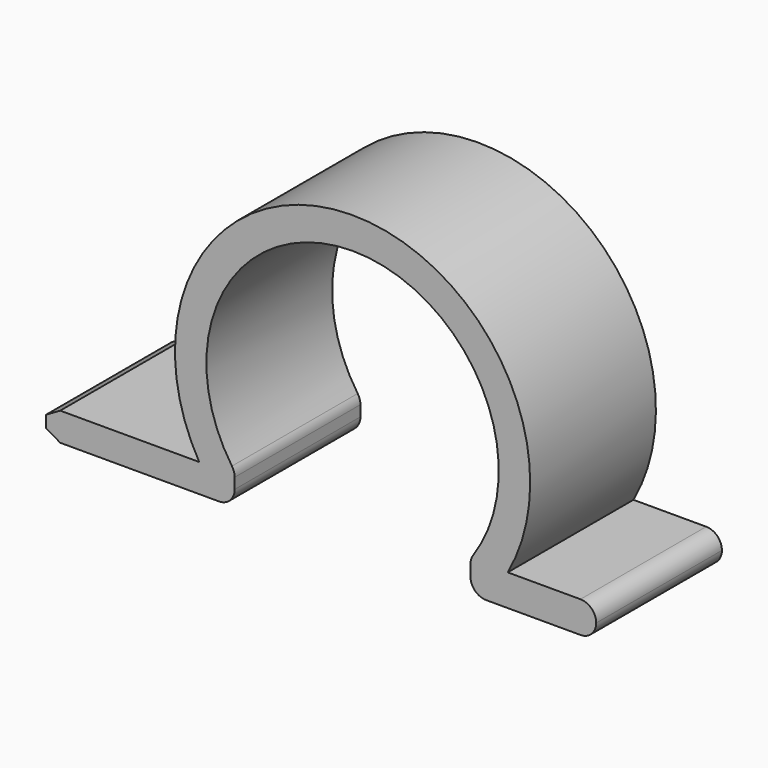
from build123d import *

# Parameters (mm, degrees)
F1_DEPTH   = 12.7
F2_SIZE2   = 0.6599113577
F2_SIZE    = 1.143
F2_2_SIZE2 = 0.6599113577
F2_2_SIZE  = 1.143
F3_R       = 1.26999


# Not quite as in the source:
# - a fillet or chamfer is up to 0.001 mm smaller than in the source, because OpenCascade refuses the exact size


with BuildPart() as f1:
    # F0 (on Front) → F1 (new body)
    with BuildSketch(Plane.XZ):
        with BuildLine():
            Line((0, 2.286), (0, 0))
            Line((0, 0), (15.24, 0))
            Line((15.24, 0), (15.24, 2.54))
            ThreePointArc((15.24, 2.54), (24.765, 21.336682776), (34.29, 2.54))
            Line((34.29, 2.54), (34.29, 0))
            Line((34.29, 0), (44.45, 0))
            Line((44.45, 0), (44.45, 2.54))
            Line((44.45, 2.54), (37.3021676826, 2.54))
            ThreePointArc((37.3021676826, 2.54), (24.6187816105, 23.8759379026), (12.3727573659, 2.286))
            Line((12.3727573659, 2.286), (0, 2.286))
        make_face()
    extrude(amount=F1_DEPTH)

    # F2
    f2_edges = [f1.edges().sort_by_distance(p)[0] for p in [
        (0, -6.35, 0),
    ]]
    f2_side = f1.faces().sort_by_distance((7.62, -6.35, 0))[0]
    chamfer(f2_edges, length=F2_SIZE, length2=F2_SIZE2, reference=f2_side)

    # F2#2
    f2_2_edges = [f1.edges().sort_by_distance(p)[0] for p in [
        (0, -6.35, 2.286),
    ]]
    f2_2_side = f1.faces().sort_by_distance((6.186379, -6.35, 2.286))[0]
    chamfer(f2_2_edges, length=F2_2_SIZE, length2=F2_2_SIZE2, reference=f2_2_side)

    # F3 (radius 1.27 in the source; OpenCascade refuses exactly that, so slightly less here)
    f3_edges = [f1.edges().sort_by_distance(p)[0] for p in [
        (44.45, -6.35, 2.54),
        (44.45, -6.35, 0),
        (34.29, -6.35, 0),
        (34.29, -6.35, 2.54),
        (15.24, -6.35, 2.54),
        (15.24, -6.35, 0),
    ]]
    fillet(f3_edges, radius=F3_R)


solid = f1.part
